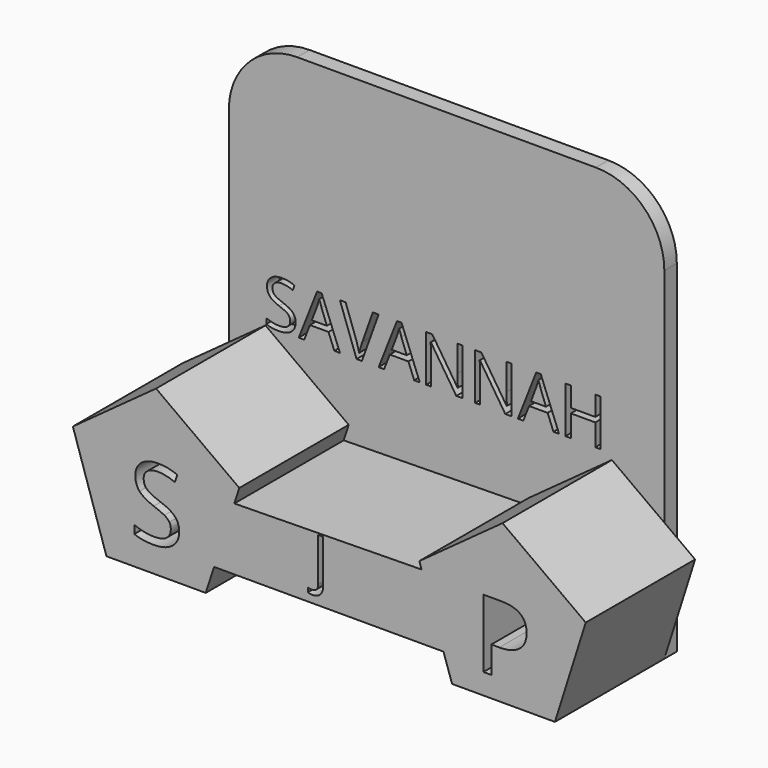
from build123d import *

# Parameters (mm, degrees)
F1_DEPTH     = 50.8
F3_DEPTH     = 152.4
F4_TEXT_SIZE = 24.1660224773
F5_DEPTH     = 5.7945984805
F6_R         = 25.4


# Not quite as in the source:
# - Text() gives the source's letters only with a copy of the font that has no kerning and outlines rounded to 1/6400 em; it was checked with that copy


with BuildPart() as f1:
    # F0 (on Front) → F1 (new body)
    with BuildSketch(Plane.XZ):
        Polygon((51.9782295413, -25.155371055), (90.1910970025, -25.155371055), (101.6340109933, 11.0664248664), (70.7191518134, 33.5273848079), (39.8042926335, 11.0664248664), (40.6384709338, 8.5844474761), (-28.9130848576, 7.5545918008), (-27.0694845462, 13.228610128), (-57.9843437262, 35.6895700695), (-88.8992029061, 13.228610128), (-76.4274913999, -25.155371055), (-39.5411960525, -25.155371055), (-36.5314893425, -15.8924462619), (-36.5314893425, -15.630371055), (48.7769319221, -15.630371055), align=None)
        with BuildLine():
            add(Edge.make_bspline(
                [(-50.9760755619, -3.9086340451), (-49.4142748891, -5.6092614444), (-49.4142748891, -8.3163826105)],
                knots=[0, 0, 0, 1, 1, 1], degree=2))
            add(Edge.make_bspline(
                [(-49.4142748891, -8.3163826105), (-49.4142748891, -11.8044041131), (-51.9449704237, -13.7595471776)],
                knots=[0, 0, 0, 1, 1, 1], degree=2))
            add(Edge.make_bspline(
                [(-51.9449704237, -13.7595471776), (-54.4756659583, -15.714690242), (-58.8140011605, -15.714690242)],
                knots=[0, 0, 0, 1, 1, 1], degree=2))
            add(Edge.make_bspline(
                [(-58.8140011605, -15.714690242), (-63.5109720727, -15.714690242), (-66.0445598308, -14.4999563854)],
                knots=[0, 0, 0, 1, 1, 1], degree=2))
            Line((-66.0445598308, -14.4999563854), (-66.0445598308, -11.538319554))
            add(Edge.make_bspline(
                [(-66.0445598308, -11.538319554), (-64.4133457948, -12.2208842925), (-62.4986938589, -12.6200111311)],
                knots=[0, 0, 0, 1, 1, 1], degree=2))
            add(Edge.make_bspline(
                [(-62.4986938589, -12.6200111311), (-60.584041923, -13.0191379697), (-58.7040966687, -13.0191379697)],
                knots=[0, 0, 0, 1, 1, 1], degree=2))
            add(Edge.make_bspline(
                [(-58.7040966687, -13.0191379697), (-55.6325553456, -13.0191379697), (-54.0765391197, -11.8535719121)],
                knots=[0, 0, 0, 1, 1, 1], degree=2))
            add(Edge.make_bspline(
                [(-54.0765391197, -11.8535719121), (-52.5205228939, -10.6880058544), (-52.5205228939, -8.6056049574)],
                knots=[0, 0, 0, 1, 1, 1], degree=2))
            add(Edge.make_bspline(
                [(-52.5205228939, -8.6056049574), (-52.5205228939, -7.2346910335), (-53.0729375763, -6.3583473226)],
                knots=[0, 0, 0, 1, 1, 1], degree=2))
            add(Edge.make_bspline(
                [(-53.0729375763, -6.3583473226), (-53.6253522587, -5.4820036118), (-54.9181761489, -4.7387021805)],
                knots=[0, 0, 0, 1, 1, 1], degree=2))
            add(Edge.make_bspline(
                [(-54.9181761489, -4.7387021805), (-56.2110000392, -3.9954007492), (-58.8487078421, -3.0583203455)],
                knots=[0, 0, 0, 1, 1, 1], degree=2))
            add(Edge.make_bspline(
                [(-58.8487078421, -3.0583203455), (-62.5334005405, -1.739466444), (-64.1154467776, 0.0681732236)],
                knots=[0, 0, 0, 1, 1, 1], degree=2))
            add(Edge.make_bspline(
                [(-64.1154467776, 0.0681732236), (-65.6974930146, 1.8758128911), (-65.6974930146, 4.7853897001)],
                knots=[0, 0, 0, 1, 1, 1], degree=2))
            add(Edge.make_bspline(
                [(-65.6974930146, 4.7853897001), (-65.6974930146, 7.8395776824), (-63.4039598044, 9.64721735)],
                knots=[0, 0, 0, 1, 1, 1], degree=2))
            add(Edge.make_bspline(
                [(-63.4039598044, 9.64721735), (-61.1104265942, 11.4548570176), (-57.3273982979, 11.4548570176)],
                knots=[0, 0, 0, 1, 1, 1], degree=2))
            add(Edge.make_bspline(
                [(-57.3273982979, 11.4548570176), (-53.3881899343, 11.4548570176), (-50.0794862868, 10.0087452835)],
                knots=[0, 0, 0, 1, 1, 1], degree=2))
            Line((-50.0794862868, 10.0087452835), (-51.0397044782, 7.336330799))
            add(Edge.make_bspline(
                [(-51.0397044782, 7.336330799), (-54.3137014441, 8.7072447229), (-57.4025961081, 8.7072447229)],
                knots=[0, 0, 0, 1, 1, 1], degree=2))
            add(Edge.make_bspline(
                [(-57.4025961081, 8.7072447229), (-59.8436327152, 8.7072447229), (-61.2174388625, 7.6602598274)],
                knots=[0, 0, 0, 1, 1, 1], degree=2))
            add(Edge.make_bspline(
                [(-61.2174388625, 7.6602598274), (-62.5912450099, 6.6132749319), (-62.5912450099, 4.7506830185)],
                knots=[0, 0, 0, 1, 1, 1], degree=2))
            add(Edge.make_bspline(
                [(-62.5912450099, 4.7506830185), (-62.5912450099, 3.3797690946), (-62.085105903, 2.5005331602)],
                knots=[0, 0, 0, 1, 1, 1], degree=2))
            add(Edge.make_bspline(
                [(-62.085105903, 2.5005331602), (-61.578966796, 1.6212972259), (-60.3758018333, 0.8895646885)],
                knots=[0, 0, 0, 1, 1, 1], degree=2))
            add(Edge.make_bspline(
                [(-60.3758018333, 0.8895646885), (-59.1726368705, 0.1578321511), (-56.6968935818, -0.7271882302)],
                knots=[0, 0, 0, 1, 1, 1], degree=2))
            add(Edge.make_bspline(
                [(-56.6968935818, -0.7271882302), (-52.5378762347, -2.2080066459), (-50.9760755619, -3.9086340451)],
                knots=[0, 0, 0, 1, 1, 1], degree=2))
        make_face(mode=Mode.SUBTRACT)
        with BuildLine():
            add(Edge.make_bspline(
                [(3.0419599349, -11.775866406), (1.9845914488, -12.9266357751), (0.0002632565, -12.9266357751)],
                knots=[0, 0, 0, 1, 1, 1], degree=2))
            add(Edge.make_bspline(
                [(0.0002632565, -12.9266357751), (-1.0324332983, -12.9266357751), (-1.6280842121, -12.630572599)],
                knots=[0, 0, 0, 1, 1, 1], degree=2))
            Line((-1.6280842121, -12.630572599), (-1.6280842121, -11.0339461849))
            add(Edge.make_bspline(
                [(-1.6280842121, -11.0339461849), (-0.8456315324, -11.2524690054), (0.0002632565, -11.2524690054)],
                knots=[0, 0, 0, 1, 1, 1], degree=2))
            add(Edge.make_bspline(
                [(0.0002632565, -11.2524690054), (1.0928773588, -11.2524690054), (1.6603317797, -10.5916137016)],
                knots=[0, 0, 0, 1, 1, 1], degree=2))
            add(Edge.make_bspline(
                [(1.6603317797, -10.5916137016), (2.2277862006, -9.9307583978), (2.2277862006, -8.6865881458)],
                knots=[0, 0, 0, 1, 1, 1], degree=2))
            Line((2.2277862006, -8.6865881458), (2.2277862006, 7.4171338976))
            Line((2.2277862006, 7.4171338976), (4.099328421, 7.4171338976))
            Line((4.099328421, 7.4171338976), (4.099328421, -8.5315074345))
            add(Edge.make_bspline(
                [(4.099328421, -8.5315074345), (4.099328421, -10.625097037), (3.0419599349, -11.775866406)],
                knots=[0, 0, 0, 1, 1, 1], degree=2))
        make_face(mode=Mode.SUBTRACT)
        with BuildLine():
            add(Edge.make_bspline(
                [(70.1831433121, 7.841417518), (79.6654317122, 7.841417518), (79.6654317122, 0.4693813846)],
                knots=[0, 0, 0, 1, 1, 1], degree=2))
            add(Edge.make_bspline(
                [(79.6654317122, 0.4693813846), (79.6654317122, -3.3744901981), (77.0428478585, -5.4432020658)],
                knots=[0, 0, 0, 1, 1, 1], degree=2))
            add(Edge.make_bspline(
                [(77.0428478585, -5.4432020658), (74.4202640049, -7.5119139334), (69.5406518084, -7.5119139334)],
                knots=[0, 0, 0, 1, 1, 1], degree=2))
            Line((69.5406518084, -7.5119139334), (66.5608205238, -7.5119139334))
            Line((66.5608205238, -7.5119139334), (66.5608205238, -17.4649935216))
            Line((66.5608205238, -17.4649935216), (63.6197602782, -17.4649935216))
            Line((63.6197602782, -17.4649935216), (63.6197602782, 7.841417518))
            Line((63.6197602782, 7.841417518), (70.1831433121, 7.841417518))
        make_face(mode=Mode.SUBTRACT)
    extrude(amount=F1_DEPTH)

    # F2 (on face) → F3 (join)
    with BuildSketch(Plane(origin=(0, 0, -25.155371055), x_dir=(1, 0, 0), z_dir=(0, 0, -1))):
        Polygon((90.1910970025, -5.7935984805), (90.1910970025, 0), (51.9782295413, 0), (-71.5900734067, 0), (-71.5900734067, -5.7935984805), align=None)
    extrude(amount=-F3_DEPTH)

    # F4 (on face) → F5 (cut, through all)
    with BuildSketch(Plane.XZ):
        with Locations((-58.8900734067, 35.6895700695)):
            Text('SAVANNAH', F4_TEXT_SIZE, font='Open Sans', text_align=(TextAlign.LEFT, TextAlign.BOTTOM))
    extrude(amount=-F5_DEPTH, mode=Mode.SUBTRACT)

    # F6
    f6_edges = [f1.edges().sort_by_distance(p)[0] for p in [
        (90.191097, 2.896799, 127.244629),
        (-71.590073, 2.896799, 127.244629),
    ]]
    fillet(f6_edges, radius=F6_R)


solid = f1.part
